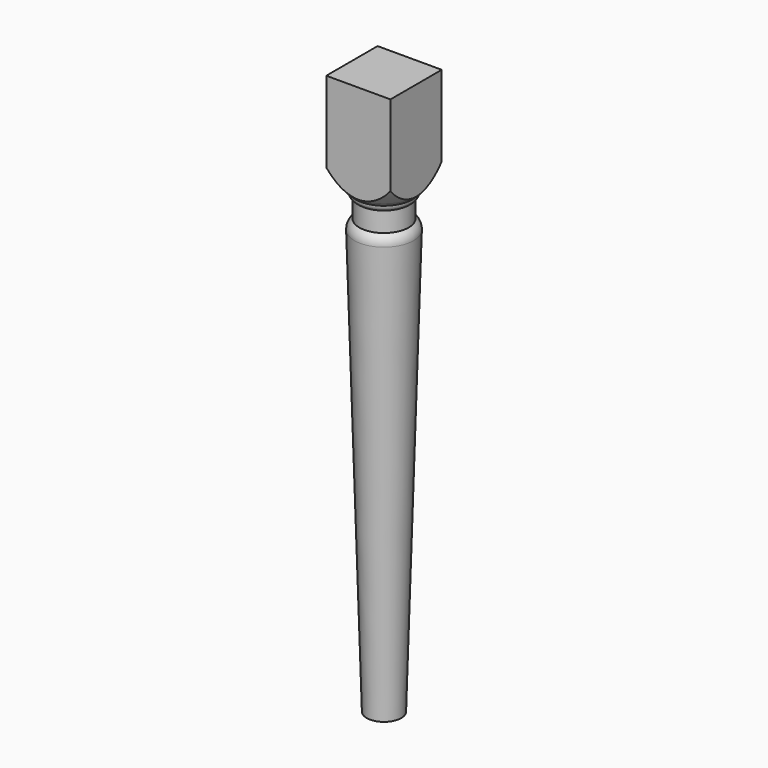
from build123d import *

# Parameters (mm, degrees)
F1_W     = 41.275
F1_H     = 89.1649350524
F1_H_2   = 37.8350649476
F2_DEPTH = 41.275
F4_DEPTH = 41.275


# Not quite as in the source:
# - a variable given as a bare number and used for a length is read in inches; the dataset says mm whatever the document's units were


with BuildPart() as f2:
    # F1 (on Front) → F2 (new body, symmetric)
    with BuildSketch(Plane.XZ):
        with Locations((20.6375, -44.5824675262)):
            Rectangle(F1_W, F1_H)
        with Locations((-20.6375, -108.0824675262)):
            Rectangle(F1_W, F1_H_2)
        with Locations((20.6375, -108.0824675262)):
            Rectangle(F1_W, F1_H_2)
    extrude(amount=F2_DEPTH, both=True)

    # F1 (on Front) → F3 (revolve, intersect)
    with BuildSketch(Plane.XZ):
        with BuildLine():
            Line((41.275, -127), (0, -127))
            Line((0, -127), (0, -723.9))
            Line((0, -723.9), (22.225, -723.9))
            Line((22.225, -723.9), (38.1, -177.8))
            ThreePointArc((38.1, -177.8), (36.5217864477, -170.6516067761), (31.75, -165.1))
            Line((31.75, -165.1), (31.75, -139.7))
            ThreePointArc((31.75, -139.7), (35.2305301109, -136.3908180665), (36.5125, -131.7625))
            ThreePointArc((36.5125, -131.7625), (38.9267731534, -129.4142731534), (41.275, -127))
        make_face()
        with Locations((20.6375, -108.0824675262)):
            Rectangle(F1_W, F1_H_2)
        with BuildLine():
            Line((41.275, -89.1649350524), (41.275, -127))
            ThreePointArc((41.275, -127), (55.2047536515, -109.2185398369), (65.6004882321, -89.1649350524))
            Line((65.6004882321, -89.1649350524), (41.275, -89.1649350524))
        make_face()
    revolve(axis=Axis((0, 0, -361.95), (0, 0, -1)), mode=Mode.INTERSECT)

    # F1 (on Front) → F4 (join, symmetric)
    with BuildSketch(Plane.XZ):
        with Locations((-20.6375, -44.5824675262)):
            Rectangle(F1_W, F1_H)
        with Locations((20.6375, -44.5824675262)):
            Rectangle(F1_W, F1_H)
    extrude(amount=F4_DEPTH, both=True)

    # F1 (on Front) → F5 (revolve)
    with BuildSketch(Plane.XZ):
        with BuildLine():
            Line((41.275, -127), (0, -127))
            Line((0, -127), (0, -723.9))
            Line((0, -723.9), (22.225, -723.9))
            Line((22.225, -723.9), (38.1, -177.8))
            ThreePointArc((38.1, -177.8), (36.5217864477, -170.6516067761), (31.75, -165.1))
            Line((31.75, -165.1), (31.75, -139.7))
            ThreePointArc((31.75, -139.7), (35.2305301109, -136.3908180665), (36.5125, -131.7625))
            ThreePointArc((36.5125, -131.7625), (38.9267731534, -129.4142731534), (41.275, -127))
        make_face()
    revolve(axis=Axis((0, 0, -361.95), (0, 0, -1)))


solid = f2.part
